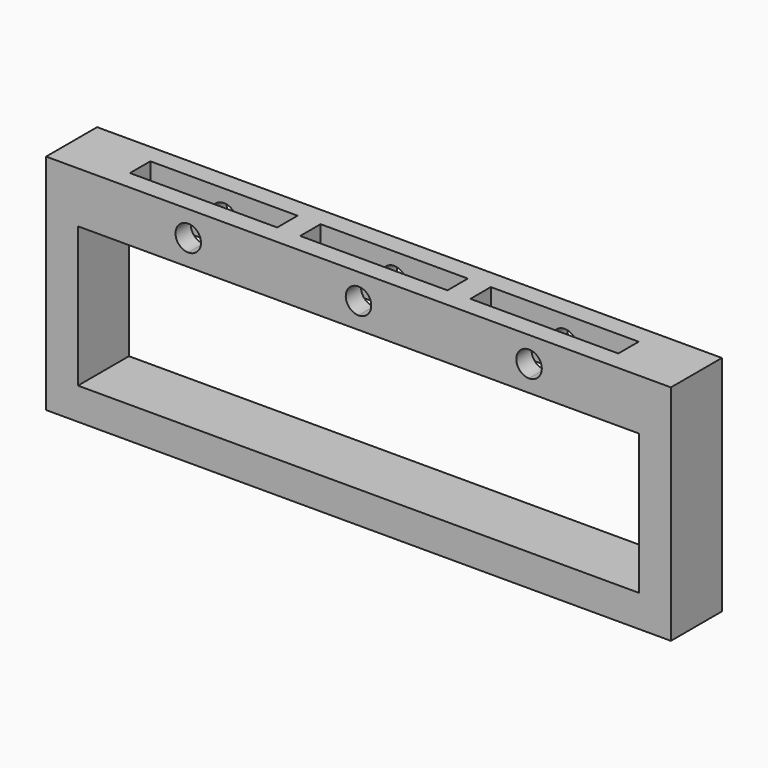
from build123d import *

# Parameters (mm, degrees)
F0_W     = 88
F0_H     = 5
F1_DEPTH = 5
F2_W     = 23.1
F2_H     = 4
F2_W_2   = 23.2
F3_DEPTH = 17.501
F5_DEPTH = 10.001


# Not quite as in the source:
# - a feature names something its author has since deleted; it is built from what else it names


with BuildPart() as f1:
    # F0 (on Front) → F1 (new body, symmetric)
    with BuildSketch(Plane.XZ):
        Polygon((44, -17.5), (49, -17.5), (49, 17.5), (-49, 17.5), (-49, -17.5), (-44, -17.5), (-44, -12.5), (-44, 9.5), (44, 9.5), (44, -12.5), align=None)
        with Locations((0, -15)):
            Rectangle(F0_W, F0_H)
    extrude(amount=F1_DEPTH, both=True)

    # F2 (on Top) → F3 (cut, through all)
    with BuildSketch(Plane.XY):
        with Locations((-26.7, 0)):
            Rectangle(F2_W, F2_H)
        Rectangle(F2_W, F2_H)
        with Locations((26.75, 0)):
            Rectangle(F2_W_2, F2_H)
    extrude(amount=F3_DEPTH, mode=Mode.SUBTRACT)

    # F4 (on face) → F5 (cut, through all)
    with BuildSketch(Plane.XZ.offset(5)):
        with BuildLine():
            ThreePointArc((-26.7, 15.5), (-28.7, 13.5), (-26.7, 11.5))
            Line((-26.7, 11.5), (-26.7, 15.5))
        make_face()
        with BuildLine():
            Line((-26.7, 15.5), (-26.7, 11.5))
            ThreePointArc((-26.7, 11.5), (-25.2857864376, 12.0857864376), (-24.7, 13.5))
            ThreePointArc((-24.7, 13.5), (-25.2857864376, 14.9142135624), (-26.7, 15.5))
        make_face()
        with BuildLine():
            ThreePointArc((0, 15.5), (-2, 13.5), (0, 11.5))
            Line((0, 11.5), (0, 15.5))
        make_face()
        with BuildLine():
            Line((0, 15.5), (0, 11.5))
            ThreePointArc((0, 11.5), (1.4142135624, 12.0857864376), (2, 13.5))
            ThreePointArc((2, 13.5), (1.4142135624, 14.9142135624), (0, 15.5))
        make_face()
        with BuildLine():
            ThreePointArc((26.75, 15.5), (24.75, 13.5), (26.75, 11.5))
            Line((26.75, 11.5), (26.75, 15.5))
        make_face()
        with BuildLine():
            Line((26.75, 15.5), (26.75, 11.5))
            ThreePointArc((26.75, 11.5), (28.1642135624, 12.0857864376), (28.75, 13.5))
            ThreePointArc((28.75, 13.5), (28.1642135624, 14.9142135624), (26.75, 15.5))
        make_face()
    extrude(amount=-F5_DEPTH, mode=Mode.SUBTRACT)


solid = f1.part
